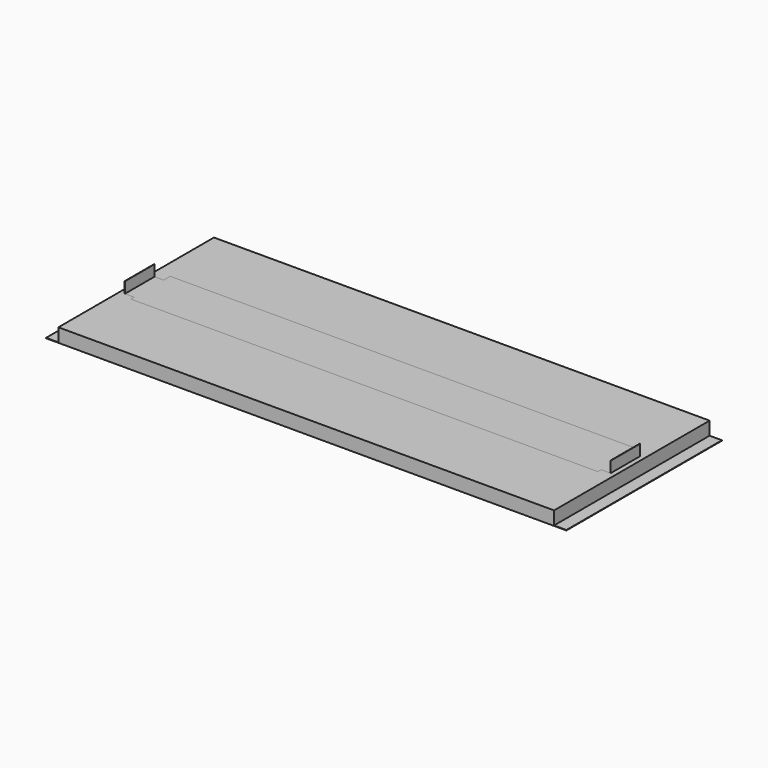
from build123d import *

# Parameters (mm, degrees)
F0_W     = 2298.7
F0_H     = 901.7
F1_DEPTH = 63.5
F2_W     = 57.15
F2_H     = 901.7
F3_DEPTH = 1.9812
F4_W     = 2254.25
F4_H     = 228.6
F5_DEPTH = 63.5
F6_W     = 44.45
F6_H     = 38.1
F6_H_2   = 19.05
F7_DEPTH = 63.501
F9_DEPTH = 1.5875


# Not quite as in the source:
# - a pattern or mirror of a feature is missing from the dataset's text; its kind, count and spacing are read off the source's solid


with BuildPart() as f1:
    # F0 (on Top) → F1 (new body)
    with BuildSketch(Plane.XY):
        Rectangle(F0_W, F0_H)
    extrude(amount=F1_DEPTH)

    # F2 (on face) → F3 (join)
    with BuildSketch(Plane(origin=(0, 0, 0), x_dir=(1, 0, 0), z_dir=(0, 0, -1))):
        with Locations((-1177.925, 0)):
            Rectangle(F2_W, F2_H)
        with Locations((1177.925, 0)):
            Rectangle(F2_W, F2_H)
    extrude(amount=-F3_DEPTH)


with BuildPart() as f5:
    # F4 (on Top) → F5 (new body)
    with BuildSketch(Plane.XY):
        Rectangle(F4_W, F4_H)
    extrude(amount=F5_DEPTH)

    # F6 (on face) → F7 (cut, through all)
    with BuildSketch(Plane.XY.offset(63.5)):
        with Locations((-1104.9, 95.25)):
            Rectangle(F6_W, F6_H)
        with Locations((-1104.9, -104.775)):
            Rectangle(F6_W, F6_H_2)
        with Locations((1104.9, -104.775)):
            Rectangle(F6_W, F6_H_2)
        with Locations((1104.9, 95.25)):
            Rectangle(F6_W, F6_H)
    extrude(amount=-F7_DEPTH, mode=Mode.SUBTRACT)

    # F8 (on face) → F9 (join)
    with BuildSketch(Plane(origin=(-1127.125, 0, 0), x_dir=(0, -1, 0), z_dir=(-1, 0, 0))):
        Polygon((-76.2, 114.3), (-76.2, 31.75), (-76.2, -50.8), (95.25, -50.8), (95.25, 31.75), (95.25, 114.3), align=None)
    f9 = extrude(amount=-F9_DEPTH)

    # F9_copies: F9 across plane
    add(f9.mirror(Plane(origin=(0, 0, 0), x_dir=(0, 0, 1), z_dir=(1, 0, 0))))


solid = Compound([f1.part, f5.part])
